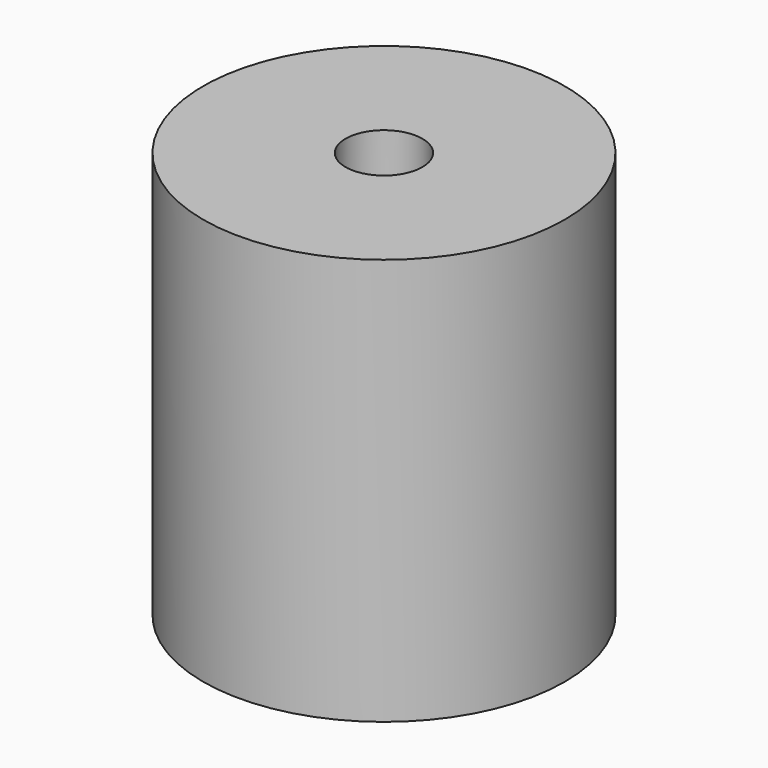
from build123d import *

# Parameters (mm, degrees)
F0_R      = 25.4
F1_DEPTH  = 38.1
F3_R      = 4.1275
F4_DEPTH  = 20.0914
F5_R      = 3.4925
F6_DEPTH  = 18.0096
F7_W      = 5.08
F7_H      = 26.67
F8_DEPTH  = 5.08
F9_R      = 25.4
F9_R_2    = 4.1275
F10_DEPTH = 6.35
F11_R     = 25.4
F11_R_2   = 5.3975
F12_DEPTH = 12.7
F13_R     = 2.54
F14_DEPTH = 25.4
F16_R     = 22.225
F16_R_2   = 6.35
F17_DEPTH = 44.45


with BuildPart() as f1:
    # F0 (on Top) → F1 (new body)
    with BuildSketch(Plane.XY):
        Circle(F0_R)
    extrude(amount=-F1_DEPTH)

    # F3 (on face) → F4 (cut)
    with BuildSketch(Plane.XY):
        Circle(F3_R)
    extrude(amount=-F4_DEPTH, mode=Mode.SUBTRACT)

    # F5 (on face) → F6 (cut, through all)
    with BuildSketch(Plane.XY.offset(-20.0914)):
        Circle(F5_R)
    extrude(amount=-F6_DEPTH, mode=Mode.SUBTRACT)

    # F7 (on face) → F8 (cut)
    with BuildSketch(Plane(origin=(0, 0, -38.1), x_dir=(1, 0, 0), z_dir=(0, 0, -1))):
        with Locations((0, -13.335)):
            Rectangle(F7_W, F7_H)
    extrude(amount=-F8_DEPTH, mode=Mode.SUBTRACT)

    # F9 (on face) → F10 (join)
    with BuildSketch(Plane.XY):
        Circle(F9_R)
        Circle(F9_R_2, mode=Mode.SUBTRACT)
    extrude(amount=F10_DEPTH)

    # F11 (on face) → F12 (join)
    with BuildSketch(Plane.XY.offset(6.35)):
        Circle(F11_R)
        Circle(F11_R_2, mode=Mode.SUBTRACT)
    extrude(amount=F12_DEPTH)

    # F13 (on offset) → F14 (cut, through all)
    with BuildSketch(Plane.XZ.offset(-25.4)):
        with Locations((0, 1.524)):
            Circle(F13_R)
    extrude(amount=F14_DEPTH, mode=Mode.SUBTRACT)

    # F16 (on offset) → F17 (cut)
    with BuildSketch(Plane(origin=(0, 0, -31.75), x_dir=(1, 0, 0), z_dir=(0, 0, -1))):
        Circle(F16_R)
        Circle(F16_R_2, mode=Mode.SUBTRACT)
    extrude(amount=-F17_DEPTH, mode=Mode.SUBTRACT)


solid = f1.part
